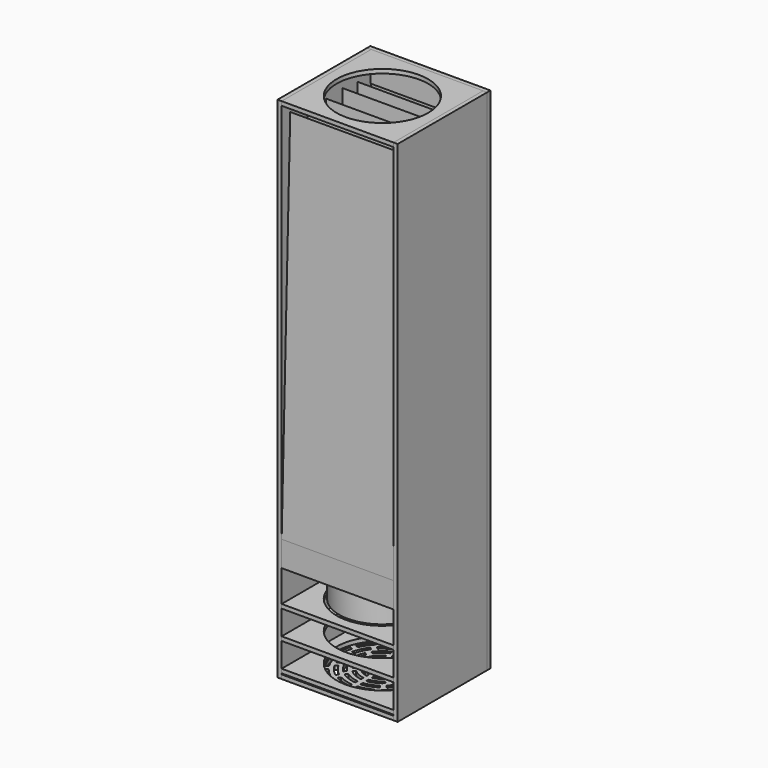
from build123d import *

# Parameters (mm, degrees)
F0_W      = 220
F0_H      = 220
F0_R      = 90
F1_DEPTH  = 8
F2_W      = 220
F2_H      = 1000
F3_DEPTH  = 8
F4_W      = 220
F4_H      = 8
F5_DEPTH  = 8
F7_DEPTH  = 220
F10_R     = 85
F10_R_2   = 43.039121025
F11_DEPTH = 51
F14_W     = 210
F14_H     = 44
F15_DEPTH = 8
F14_H_2   = 59
F17_R     = 90
F18_DEPTH = 8


# Not quite as in the source:
# - a feature names something its author has since deleted; it is built from what else it names


with BuildPart() as f1:
    # F0 (on Top) → F1 (new body)
    with BuildSketch(Plane.XY):
        with Locations((5.6901878119, 12.2554755211)):
            Rectangle(F0_W, F0_H)
        with Locations((5.6901878119, 12.2554755211)):
            Circle(F0_R, mode=Mode.SUBTRACT)
    extrude(amount=F1_DEPTH)


with BuildPart() as f3:
    # F2 (on face) → F3 (new body)
    with BuildSketch(Plane(origin=(-104.3098121881, 0, 0), x_dir=(0, -1, 0), z_dir=(-1, 0, 0))):
        with Locations((-12.2554755211, -492)):
            Rectangle(F2_W, F2_H)
    extrude(amount=F3_DEPTH)


with BuildPart() as f5:
    # F4 (on face) → F5 (new body)
    with BuildSketch(Plane(origin=(0, 122.2554755211, 0), x_dir=(-1, 0, 0), z_dir=(0, 1, 0))):
        with Locations((-5.6901878119, 4)):
            Rectangle(F4_W, F4_H)
        Polygon((-115.6901878119, 8), (-123.6901878119, 8), (-123.6901878119, -992), (112.3098121881, -992), (112.3098121881, 8), (104.3098121881, 8), (104.3098121881, 0), (-115.6901878119, 0), align=None)
    extrude(amount=F5_DEPTH)


with BuildPart() as f7:
    # F6 (on face) → F7 (new body)
    with BuildSketch(Plane.YZ.offset(-104.3098121881)):
        Polygon((-97.7445244789, -800), (122.2554755211, -800), (122.2554755211, -750), (107.9942195405, -750), (88.9521464705, -34.4358831644), (71.1688101292, -750), (52.0175285637, -30.3320400417), (34.2342145741, -750), (10.9790684655, -31.699988991), (-17.7478455007, -750), (-32.7952764928, -23.492295295), (-64.2581060529, -750), (-76.5696465969, -19.3884503096), (-97.7445244789, -750), align=None)
    extrude(amount=F7_DEPTH)


with BuildPart() as f8_1:
    # F8: copy of F1
    add(f1.part.moved(Location((0, 0, -870))))


with BuildPart() as f9_1:
    # F9: copy of F8_1
    add(f8_1.part.moved(Location((0, 0, -122))))


with BuildPart() as f11:
    # F10 (on face) → F11 (new body)
    with BuildSketch(Plane.XY.offset(-862)):
        with Locations((5.6901878119, 12.2554755211)):
            Circle(F10_R)
        with Locations((5.6901878119, 12.2554755211)):
            Circle(F10_R_2, mode=Mode.SUBTRACT)
    extrude(amount=F11_DEPTH)


with BuildPart() as f12_1:
    # F12: copy of F9_1
    add(f9_1.part.moved(Location((0, 0, 10))))


with BuildPart() as f13_1:
    # F13: copy of F12_1
    add(f12_1.part.moved(Location((0, 0, 56))))


with BuildPart() as f15:
    # F14 (on face) → F15 (new body)
    with BuildSketch(Plane.XZ.offset(-122.2554755211)):
        with Locations((5.6901878119, -950)):
            Rectangle(F14_W, F14_H)
    extrude(amount=F15_DEPTH)


with BuildPart() as f15b:
    # F14 (on face) → F15, piece 2 (new body)
    with BuildSketch(Plane.XZ.offset(-122.2554755211)):
        with Locations((5.6901878119, -894)):
            Rectangle(F14_W, F14_H)
    extrude(amount=F15_DEPTH)


with BuildPart() as f15c:
    # F14 (on face) → F15, piece 3 (new body)
    with BuildSketch(Plane.XZ.offset(-122.2554755211)):
        with Locations((5.6901878119, -830.5)):
            Rectangle(F14_W, F14_H_2)
    extrude(amount=F15_DEPTH)


with BuildPart() as f15d:
    # F14 (on face) → F15, piece 4 (new body)
    with BuildSketch(Plane.XZ.offset(-122.2554755211)):
        with Locations((5.6901878119, -726)):
            Rectangle(F14_W, F14_H)
    extrude(amount=F15_DEPTH)


with BuildPart() as f15e:
    # F14 (on face) → F15, piece 5 (new body)
    with BuildSketch(Plane.XZ.offset(-122.2554755211)):
        with Locations((5.6901878119, -24)):
            Rectangle(F14_W, F14_H)
    extrude(amount=F15_DEPTH)


with BuildPart() as f16_1:
    # F16: copy of F3
    add(f3.part.moved(Location((228, 0, 0))))


with BuildPart() as f9_1_1:
    add(f9_1.part)

    # F17 (on face) → F18 (join)
    with BuildSketch(Plane(origin=(0, 0, -992), x_dir=(1, 0, 0), z_dir=(0, 0, -1))):
        with Locations((5.6901878119, -12.2554755211)):
            Circle(F17_R)
        with BuildLine():
            Line((-10.6007107267, -99.2431564007), (-9.1623520978, -93.4075060455))
            ThreePointArc((-9.1623520978, -93.4075060455), (5.6901878119, -94.7554755211), (20.5427277215, -93.4075060455))
            Line((20.5427277215, -93.4075060455), (21.9810863504, -99.2431564007))
            ThreePointArc((21.9810863504, -99.2431564007), (5.6901878119, -100.7554755211), (-10.6007107267, -99.2431564007))
        make_face(mode=Mode.SUBTRACT)
        with BuildLine():
            Line((-49.1598774495, -81.7084836692), (-45.1743121905, -77.2097104832))
            ThreePointArc((-45.1743121905, -77.2097104832), (-32.6494738818, -85.3055976375), (-18.871770272, -91.0143494026))
            Line((-18.871770272, -91.0143494026), (-20.310128901, -96.8499997578))
            ThreePointArc((-20.310128901, -96.8499997578), (-35.437812914, -90.6183337914), (-49.1598774495, -81.7084836692))
        make_face(mode=Mode.SUBTRACT)
        with BuildLine():
            ThreePointArc((-20.0490286272, -82.1678688223), (-34.5875530886, -74.928863717), (-47.211905075, -64.7113481017))
            Line((-47.211905075, -64.7113481017), (-42.6662596699, -60.7725239365))
            ThreePointArc((-42.6662596699, -60.7725239365), (-31.3437081839, -69.88134252), (-18.3544774876, -76.3967576305))
            Line((-18.3544774876, -76.3967576305), (-20.0490286272, -82.1678688223))
        make_face(mode=Mode.SUBTRACT)
        with BuildLine():
            Line((-75.1535552359, -48.2629637705), (-69.5338283163, -46.1316824745))
            ThreePointArc((-69.5338283163, -46.1316824745), (-62.2059811244, -59.1208171264), (-52.6594196722, -70.5784839008))
            Line((-52.6594196722, -70.5784839008), (-56.6449849312, -75.0772570868))
            ThreePointArc((-56.6449849312, -75.0772570868), (-67.1438843197, -62.5292056068), (-75.1535552359, -48.2629637705))
        make_face(mode=Mode.SUBTRACT)
        with BuildLine():
            Line((-67.1736705557, -27.7831329038), (-61.2201411832, -26.9271446073))
            ThreePointArc((-61.2201411832, -26.9271446073), (-56.6196038699, -40.7114039117), (-49.2148670093, -53.215028193))
            Line((-49.2148670093, -53.215028193), (-53.7605124145, -57.1538523581))
            ThreePointArc((-53.7605124145, -57.1538523581), (-62.0773958421, -43.2038939897), (-67.1736705557, -27.7831329038))
        make_face(mode=Mode.SUBTRACT)
        with BuildLine():
            Line((-82.6269057627, -6.5685622512), (-76.6604288949, -7.2930237053))
            ThreePointArc((-76.6604288949, -7.2930237053), (-76.2082943012, -22.1997516422), (-73.0798771867, -36.7815200476))
            Line((-73.0798771867, -36.7815200476), (-78.6996041063, -38.9128013437))
            ThreePointArc((-78.6996041063, -38.9128013437), (-82.1645475458, -22.9229717237), (-82.6269057627, -6.5685622512))
        make_face(mode=Mode.SUBTRACT)
        with BuildLine():
            Line((-44.0251116702, -46.7321197518), (-38.8091472898, -43.7206813127))
            ThreePointArc((-38.8091472898, -43.7206813127), (-29.3417369161, -54.0048976711), (-17.5697623541, -61.5426413787))
            Line((-17.5697623541, -61.5426413787), (-19.6297075672, -67.2022943371))
            ThreePointArc((-19.6297075672, -67.2022943371), (-33.1984625742, -58.6011643298), (-44.0251116702, -46.7321197518))
        make_face(mode=Mode.SUBTRACT)
        with BuildLine():
            Line((-38.2685160911, -27.417347146), (-32.3797289015, -26.0732698978))
            ThreePointArc((-32.3797289015, -26.0732698978), (-25.9739872281, -37.5068124964), (-16.2525190335, -46.2961514294))
            Line((-16.2525190335, -46.2961514294), (-18.8732758842, -51.738209105))
            ThreePointArc((-18.8732758842, -51.738209105), (-30.6649761229, -41.2477513075), (-38.2685160911, -27.417347146))
        make_face(mode=Mode.SUBTRACT)
        with BuildLine():
            Line((-54.5551008294, -6.7097387325), (-48.6237249844, -7.7556003267))
            ThreePointArc((-48.6237249844, -7.7556003267), (-47.9818347273, -21.7193012039), (-43.8091472898, -35.0604272749))
            Line((-43.8091472898, -35.0604272749), (-49.0251116702, -38.0718657139))
            ThreePointArc((-49.0251116702, -38.0718657139), (-53.8906812454, -22.7611902699), (-54.5551008294, -6.7097387325))
        make_face(mode=Mode.SUBTRACT)
        with BuildLine():
            Line((-26.3962525282, -7.0872701938), (-20.6052179604, -8.9688913864))
            ThreePointArc((-20.6052179604, -8.9688913864), (-19.51280987, -20.444425872), (-13.6514366471, -30.3704296554))
            Line((-13.6514366471, -30.3704296554), (-17.23049284, -35.2965778917))
            ThreePointArc((-17.23049284, -35.2965778917), (-25.2191489677, -22.2985278383), (-26.3962525282, -7.0872701938))
        make_face(mode=Mode.SUBTRACT)
        with BuildLine():
            Line((-10.4540988911, -84.9851943907), (-8.7595477515, -79.2140831989))
            ThreePointArc((-8.7595477515, -79.2140831989), (5.6901878119, -80.7554755211), (20.1399233752, -79.2140831989))
            Line((20.1399233752, -79.2140831989), (21.8344745148, -84.9851943907))
            ThreePointArc((21.8344745148, -84.9851943907), (5.6901878119, -86.7554755211), (-10.4540988911, -84.9851943907))
        make_face(mode=Mode.SUBTRACT)
        with BuildLine():
            Line((-10.2327813593, -70.6224957703), (-8.1728361462, -64.962842812))
            ThreePointArc((-8.1728361462, -64.962842812), (5.6901878119, -66.7554755211), (19.5532117699, -64.962842812))
            Line((19.5532117699, -64.962842812), (21.613156983, -70.6224957703))
            ThreePointArc((21.613156983, -70.6224957703), (5.6901878119, -72.7554755211), (-10.2327813593, -70.6224957703))
        make_face(mode=Mode.SUBTRACT)
        with BuildLine():
            Line((31.6905045247, -96.8499997578), (30.2521458957, -91.0143494026))
            ThreePointArc((30.2521458957, -91.0143494026), (44.0298495055, -85.3055976375), (56.5546878142, -77.2097104832))
            Line((56.5546878142, -77.2097104832), (60.5402530732, -81.7084836692))
            ThreePointArc((60.5402530732, -81.7084836692), (46.8181885377, -90.6183337914), (31.6905045247, -96.8499997578))
        make_face(mode=Mode.SUBTRACT)
        with BuildLine():
            Line((31.4294042509, -82.1678688223), (29.7348531113, -76.3967576305))
            ThreePointArc((29.7348531113, -76.3967576305), (42.7240838076, -69.88134252), (54.0466352936, -60.7725239365))
            Line((54.0466352936, -60.7725239365), (58.5922806987, -64.7113481017))
            ThreePointArc((58.5922806987, -64.7113481017), (45.9679287123, -74.928863717), (31.4294042509, -82.1678688223))
        make_face(mode=Mode.SUBTRACT)
        with BuildLine():
            Line((-9.8635872051, -56.0770464961), (-7.2428303545, -50.6349888206))
            ThreePointArc((-7.2428303545, -50.6349888206), (5.6901878119, -52.7554755211), (18.6232059782, -50.6349888206))
            Line((18.6232059782, -50.6349888206), (21.2439628288, -56.0770464961))
            ThreePointArc((21.2439628288, -56.0770464961), (5.6901878119, -58.7554755211), (-9.8635872051, -56.0770464961))
        make_face(mode=Mode.SUBTRACT)
        with BuildLine():
            Line((-9.1403228963, -41.1744304146), (-5.5612667034, -36.2482821783))
            ThreePointArc((-5.5612667034, -36.2482821783), (5.6901878119, -38.7554755211), (16.9416423271, -36.2482821783))
            Line((16.9416423271, -36.2482821783), (20.52069852, -41.1744304146))
            ThreePointArc((20.52069852, -41.1744304146), (5.6901878119, -44.7554755211), (-9.1403228963, -41.1744304146))
        make_face(mode=Mode.SUBTRACT)
        with BuildLine():
            Line((31.0100831909, -67.2022943371), (28.9501379778, -61.5426413787))
            ThreePointArc((28.9501379778, -61.5426413787), (40.7221125398, -54.0048976711), (50.1895229135, -43.7206813127))
            Line((50.1895229135, -43.7206813127), (55.4054872939, -46.7321197518))
            ThreePointArc((55.4054872939, -46.7321197518), (44.5788381979, -58.6011643298), (31.0100831909, -67.2022943371))
        make_face(mode=Mode.SUBTRACT)
        with BuildLine():
            Line((-7.2350350391, -25.4913591053), (-1.7313796046, -22.3138221587))
            ThreePointArc((-1.7313796046, -22.3138221587), (5.6901878119, -24.7554755211), (13.1117552283, -22.3138221587))
            Line((13.1117552283, -22.3138221587), (18.6154106628, -25.4913591053))
            ThreePointArc((18.6154106628, -25.4913591053), (5.6901878119, -30.7554755211), (-7.2350350391, -25.4913591053))
        make_face(mode=Mode.SUBTRACT)
        with BuildLine():
            Line((28.6108684637, -35.2965778917), (25.0318122708, -30.3704296554))
            ThreePointArc((25.0318122708, -30.3704296554), (30.8931854937, -20.444425872), (31.9855935841, -8.9688913864))
            Line((31.9855935841, -8.9688913864), (37.7766281519, -7.0872701938))
            ThreePointArc((37.7766281519, -7.0872701938), (36.5995245914, -22.2985278383), (28.6108684637, -35.2965778917))
        make_face(mode=Mode.SUBTRACT)
        with BuildLine():
            Line((30.2536515079, -51.738209105), (27.6328946572, -46.2961514294))
            ThreePointArc((27.6328946572, -46.2961514294), (37.3543628518, -37.5068124964), (43.7601045252, -26.0732698978))
            Line((43.7601045252, -26.0732698978), (49.6488917148, -27.417347146))
            ThreePointArc((49.6488917148, -27.417347146), (42.0453517466, -41.2477513075), (30.2536515079, -51.738209105))
        make_face(mode=Mode.SUBTRACT)
        with BuildLine():
            Line((60.4054872939, -38.0718657139), (55.1895229135, -35.0604272749))
            ThreePointArc((55.1895229135, -35.0604272749), (59.362210351, -21.7193012039), (60.0041006081, -7.7556003267))
            Line((60.0041006081, -7.7556003267), (65.9354764531, -6.7097387325))
            ThreePointArc((65.9354764531, -6.7097387325), (65.2710568691, -22.7611902699), (60.4054872939, -38.0718657139))
        make_face(mode=Mode.SUBTRACT)
        with BuildLine():
            Line((68.0253605549, -75.0772570868), (64.0397952959, -70.5784839008))
            ThreePointArc((64.0397952959, -70.5784839008), (73.5863567481, -59.1208171264), (80.91420394, -46.1316824745))
            Line((80.91420394, -46.1316824745), (86.5339308596, -48.2629637705))
            ThreePointArc((86.5339308596, -48.2629637705), (78.5242599434, -62.5292056068), (68.0253605549, -75.0772570868))
        make_face(mode=Mode.SUBTRACT)
        with BuildLine():
            Line((65.1408880382, -57.1538523581), (60.5952426331, -53.215028193))
            ThreePointArc((60.5952426331, -53.215028193), (67.9999794936, -40.7114039117), (72.6005168069, -26.9271446073))
            Line((72.6005168069, -26.9271446073), (78.5540461794, -27.7831329038))
            ThreePointArc((78.5540461794, -27.7831329038), (73.4577714658, -43.2038939897), (65.1408880382, -57.1538523581))
        make_face(mode=Mode.SUBTRACT)
        with BuildLine():
            Line((90.07997973, -38.9128013437), (84.4602528104, -36.7815200476))
            ThreePointArc((84.4602528104, -36.7815200476), (87.5886699249, -22.1997516422), (88.0408045186, -7.2930237053))
            Line((88.0408045186, -7.2930237053), (94.0072813864, -6.5685622512))
            ThreePointArc((94.0072813864, -6.5685622512), (93.5449231695, -22.9229717237), (90.07997973, -38.9128013437))
        make_face(mode=Mode.SUBTRACT)
        with BuildLine():
            Line((-64.0016758361, 14.0750038), (-58.5304660063, 11.5763859917))
            ThreePointArc((-58.5304660063, 11.5763859917), (-62.112580957, -2.5069090994), (-62.6432895659, -17.0289301885))
            Line((-62.6432895659, -17.0289301885), (-68.5968189384, -17.8849184849))
            ThreePointArc((-68.5968189384, -17.8849184849), (-68.0515096083, -1.6530200697), (-64.0016758361, 14.0750038))
        make_face(mode=Mode.SUBTRACT)
        with BuildLine():
            Line((-69.867874488, 33.8230359728), (-64.9214956184, 30.4087971569))
            ThreePointArc((-64.9214956184, 30.4087971569), (-71.4486522097, 16.9994276599), (-75.4550620923, 2.6340650357))
            Line((-75.4550620923, 2.6340650357), (-81.4215389602, 3.3585264898))
            ThreePointArc((-81.4215389602, 3.3585264898), (-77.0587496658, 19.1270569822), (-69.867874488, 33.8230359728))
        make_face(mode=Mode.SUBTRACT)
        with BuildLine():
            Line((-33.5716443441, 12.6595507836), (-28.8492036786, 8.8935300223))
            ThreePointArc((-28.8492036786, 8.8935300223), (-33.7943926315, -3.2433776959), (-34.6049382411, -16.323990776))
            Line((-34.6049382411, -16.323990776), (-40.4937254307, -17.6680680241))
            ThreePointArc((-40.4937254307, -17.6680680241), (-39.6439601046, -1.9082520921), (-33.5716443441, 12.6595507836))
        make_face(mode=Mode.SUBTRACT)
        with BuildLine():
            Line((0.6901878119, 5.5560376095), (0.6901878119, -0.7990362837))
            ThreePointArc((0.6901878119, -0.7990362837), (-5.1351297355, -6.0054755211), (-6.7313796046, -13.6535681209))
            Line((-6.7313796046, -13.6535681209), (-12.2350350391, -16.8311050674))
            ThreePointArc((-12.2350350391, -16.8311050674), (-10.3312821582, -3.0054755211), (0.6901878119, 5.5560376095))
        make_face(mode=Mode.SUBTRACT)
        with BuildLine():
            Line((0.6901878119, 19.8576059256), (0.6901878119, 13.7685518383))
            ThreePointArc((0.6901878119, 13.7685518383), (-9.8861213739, 9.1834748298), (-17.5150480166, 0.5416737765))
            Line((-17.5150480166, 0.5416737765), (-23.3060825844, 2.4232949692))
            ThreePointArc((-23.3060825844, 2.4232949692), (-13.4128328877, 14.0375767961), (0.6901878119, 19.8576059256))
        make_face(mode=Mode.SUBTRACT)
        with BuildLine():
            Line((-36.8956498816, 30.7177304094), (-33.0242192496, 26.1039390453))
            ThreePointArc((-33.0242192496, 26.1039390453), (-41.5081966944, 14.9945244789), (-46.8872432077, 2.0924772034))
            Line((-46.8872432077, 2.0924772034), (-52.8186190528, 3.1383387976))
            ThreePointArc((-52.8186190528, 3.1383387976), (-46.7043491171, 17.9945244789), (-36.8956498816, 30.7177304094))
        make_face(mode=Mode.SUBTRACT)
        with BuildLine():
            Line((-38.7030068274, 47.5733993615), (-35.4511870037, 42.5134689483))
            ThreePointArc((-35.4511870037, 42.5134689483), (-46.0786580314, 32.6024847542), (-54.3763158763, 20.6727059452))
            Line((-54.3763158763, 20.6727059452), (-59.8475257061, 23.1713237535))
            ThreePointArc((-59.8475257061, 23.1713237535), (-50.6131554775, 36.5316491578), (-38.7030068274, 47.5733993615))
        make_face(mode=Mode.SUBTRACT)
        with BuildLine():
            Line((0.6901878119, 33.9749257318), (0.6901878119, 27.9346974071))
            ThreePointArc((0.6901878119, 27.9346974071), (-11.8821036224, 24.233763629), (-22.61430566, 16.7118448469))
            Line((-22.61430566, 16.7118448469), (-27.3367463255, 20.4778656082))
            ThreePointArc((-27.3367463255, 20.4778656082), (-14.4854060571, 29.6395768364), (0.6901878119, 33.9749257318))
        make_face(mode=Mode.SUBTRACT)
        with BuildLine():
            Line((0.6901878119, 48.0375589025), (0.6901878119, 42.0146820243))
            ThreePointArc((0.6901878119, 42.0146820243), (-12.9499099994, 38.9577723117), (-25.3637748185, 32.5318151422))
            Line((-25.3637748185, 32.5318151422), (-29.2352054504, 37.1456065063))
            ThreePointArc((-29.2352054504, 37.1456065063), (-15.0020308594, 44.5959280365), (0.6901878119, 48.0375589025))
        make_face(mode=Mode.SUBTRACT)
        with BuildLine():
            Line((-39.7994017137, 63.6586025198), (-37.0062766311, 58.3367473088))
            ThreePointArc((-37.0062766311, 58.3367473088), (-49.017431493, 49.496661203), (-59.2408481511, 38.6386358158))
            Line((-59.2408481511, 38.6386358158), (-64.1872270207, 42.0528746317))
            ThreePointArc((-64.1872270207, 42.0528746317), (-52.9961674425, 53.9877256921), (-39.7994017137, 63.6586025198))
        make_face(mode=Mode.SUBTRACT)
        with BuildLine():
            Line((0.6901878119, 62.0765498785), (0.6901878119, 56.0617990147))
            ThreePointArc((0.6901878119, 56.0617990147), (-13.6084923318, 53.4697931715), (-27.0386516754, 47.9198771228))
            Line((-27.0386516754, 47.9198771228), (-30.2904714991, 52.9798075361))
            ThreePointArc((-30.2904714991, 52.9798075361), (-15.2988876728, 59.2267510132), (0.6901878119, 62.0765498785))
        make_face(mode=Mode.SUBTRACT)
        with BuildLine():
            Line((0.6901878119, 76.1031686514), (0.6901878119, 70.0928699389))
            ThreePointArc((0.6901878119, 70.0928699389), (-14.0533544919, 67.8472244166), (-28.1517163746, 62.9839790293))
            Line((-28.1517163746, 62.9839790293), (-30.9448414572, 68.3058342402))
            ThreePointArc((-30.9448414572, 68.3058342402), (-15.4892484776, 73.6728753211), (0.6901878119, 76.1031686514))
        make_face(mode=Mode.SUBTRACT)
        with BuildLine():
            Line((23.6154106628, -16.8311050674), (18.1117552283, -13.6535681209))
            ThreePointArc((18.1117552283, -13.6535681209), (16.5155053592, -6.0054755211), (10.6901878119, -0.7990362837))
            Line((10.6901878119, -0.7990362837), (10.6901878119, 5.5560376095))
            ThreePointArc((10.6901878119, 5.5560376095), (21.7116577819, -3.0054755211), (23.6154106628, -16.8311050674))
        make_face(mode=Mode.SUBTRACT)
        with BuildLine():
            ThreePointArc((28.8954236403, 0.5416737765), (21.2664969976, 9.1834748298), (10.6901878119, 13.7685518383))
            Line((10.6901878119, 13.7685518383), (10.6901878119, 19.8576059256))
            ThreePointArc((10.6901878119, 19.8576059256), (24.7932085114, 14.0375767961), (34.6864582081, 2.4232949692))
            Line((34.6864582081, 2.4232949692), (28.8954236403, 0.5416737765))
        make_face(mode=Mode.SUBTRACT)
        with BuildLine():
            Line((51.8741010544, -17.6680680241), (45.9853138648, -16.323990776))
            ThreePointArc((45.9853138648, -16.323990776), (45.1747682552, -3.2433776959), (40.2295793023, 8.8935300223))
            Line((40.2295793023, 8.8935300223), (44.9520199678, 12.6595507836))
            ThreePointArc((44.9520199678, 12.6595507836), (51.0243357283, -1.9082520921), (51.8741010544, -17.6680680241))
        make_face(mode=Mode.SUBTRACT)
        with BuildLine():
            ThreePointArc((33.9946812837, 16.7118448469), (23.2624792461, 24.233763629), (10.6901878119, 27.9346974071))
            Line((10.6901878119, 27.9346974071), (10.6901878119, 33.9749257318))
            ThreePointArc((10.6901878119, 33.9749257318), (25.8657816808, 29.6395768364), (38.7171219492, 20.4778656082))
            Line((38.7171219492, 20.4778656082), (33.9946812837, 16.7118448469))
        make_face(mode=Mode.SUBTRACT)
        with BuildLine():
            ThreePointArc((36.7441504422, 32.5318151422), (24.3302856231, 38.9577723117), (10.6901878119, 42.0146820243))
            Line((10.6901878119, 42.0146820243), (10.6901878119, 48.0375589025))
            ThreePointArc((10.6901878119, 48.0375589025), (26.3824064831, 44.5959280365), (40.6155810741, 37.1456065063))
            Line((40.6155810741, 37.1456065063), (36.7441504422, 32.5318151422))
        make_face(mode=Mode.SUBTRACT)
        with BuildLine():
            Line((64.1989946765, 3.1383387976), (58.2676188314, 2.0924772034))
            ThreePointArc((58.2676188314, 2.0924772034), (52.8885723181, 14.9945244789), (44.4045948734, 26.1039390453))
            Line((44.4045948734, 26.1039390453), (48.2760255053, 30.7177304094))
            ThreePointArc((48.2760255053, 30.7177304094), (58.0847247408, 17.9945244789), (64.1989946765, 3.1383387976))
        make_face(mode=Mode.SUBTRACT)
        with BuildLine():
            Line((71.2279013298, 23.1713237535), (65.7566915, 20.6727059452))
            ThreePointArc((65.7566915, 20.6727059452), (57.4590336551, 32.6024847542), (46.8315626274, 42.5134689483))
            Line((46.8315626274, 42.5134689483), (50.0833824512, 47.5733993615))
            ThreePointArc((50.0833824512, 47.5733993615), (61.9935311012, 36.5316491578), (71.2279013298, 23.1713237535))
        make_face(mode=Mode.SUBTRACT)
        with BuildLine():
            Line((79.9771945621, -17.8849184849), (74.0236651896, -17.0289301885))
            ThreePointArc((74.0236651896, -17.0289301885), (73.4929565807, -2.5069090994), (69.91084163, 11.5763859917))
            Line((69.91084163, 11.5763859917), (75.3820514598, 14.0750038))
            ThreePointArc((75.3820514598, 14.0750038), (79.431885232, -1.6530200697), (79.9771945621, -17.8849184849))
        make_face(mode=Mode.SUBTRACT)
        with BuildLine():
            Line((92.8019145839, 3.3585264898), (86.835437716, 2.6340650357))
            ThreePointArc((86.835437716, 2.6340650357), (82.8290278334, 16.9994276599), (76.3018712421, 30.4087971569))
            Line((76.3018712421, 30.4087971569), (81.2482501117, 33.8230359728))
            ThreePointArc((81.2482501117, 33.8230359728), (88.4391252895, 19.1270569822), (92.8019145839, 3.3585264898))
        make_face(mode=Mode.SUBTRACT)
        with BuildLine():
            ThreePointArc((38.4190272991, 47.9198771228), (24.9888679555, 53.4697931715), (10.6901878119, 56.0617990147))
            Line((10.6901878119, 56.0617990147), (10.6901878119, 62.0765498785))
            ThreePointArc((10.6901878119, 62.0765498785), (26.6792632965, 59.2267510132), (41.6708471228, 52.9798075361))
            Line((41.6708471228, 52.9798075361), (38.4190272991, 47.9198771228))
        make_face(mode=Mode.SUBTRACT)
        with BuildLine():
            ThreePointArc((39.5320919983, 62.9839790293), (25.4337301156, 67.8472244166), (10.6901878119, 70.0928699389))
            Line((10.6901878119, 70.0928699389), (10.6901878119, 76.1031686514))
            ThreePointArc((10.6901878119, 76.1031686514), (26.8696241013, 73.6728753211), (42.3252170809, 68.3058342402))
            Line((42.3252170809, 68.3058342402), (39.5320919983, 62.9839790293))
        make_face(mode=Mode.SUBTRACT)
        with BuildLine():
            Line((75.5676026444, 42.0528746317), (70.6212237748, 38.6386358158))
            ThreePointArc((70.6212237748, 38.6386358158), (60.3978071167, 49.496661203), (48.3866522548, 58.3367473088))
            Line((48.3866522548, 58.3367473088), (51.1797773374, 63.6586025198))
            ThreePointArc((51.1797773374, 63.6586025198), (64.3765430662, 53.9877256921), (75.5676026444, 42.0528746317))
        make_face(mode=Mode.SUBTRACT)
    extrude(amount=-F18_DEPTH)


solid = Compound([f1.part, f3.part, f5.part, f7.part, f8_1.part, f11.part, f12_1.part, f13_1.part, f15.part, f15b.part, f15c.part, f15d.part, f15e.part, f16_1.part, f9_1_1.part])
